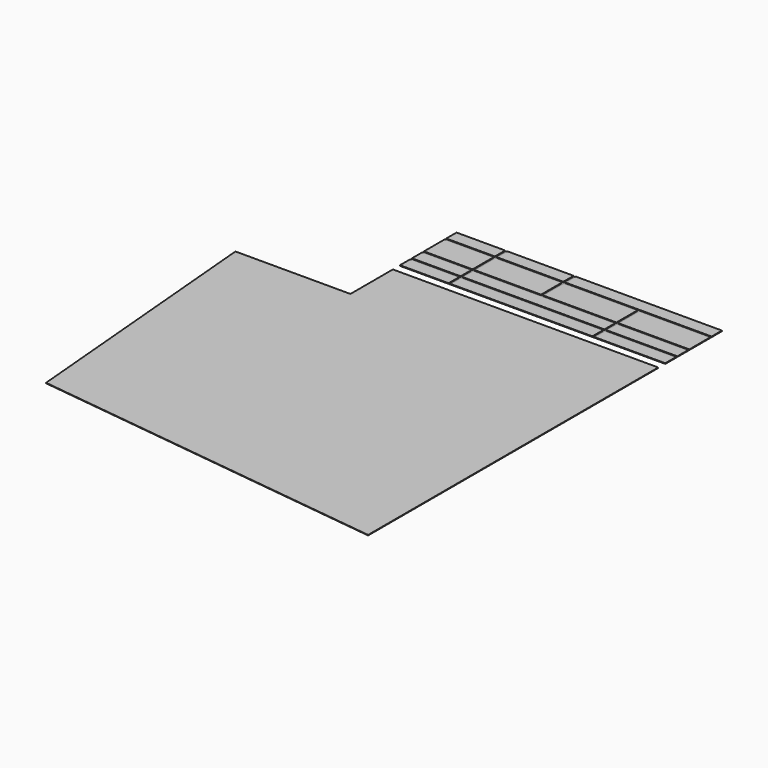
from build123d import *

# Parameters (mm, degrees)
F0_W     = 80100
F0_H     = 7280
F0_W_2   = 37500
F0_H_2   = 14560
F0_W_3   = 41400
F3_DEPTH = 25
F4_START = 280
F0_W_4   = 27500
F4_DEPTH = 70
F0_W_5   = 40000
F5_START = 280
F5_DEPTH = 70
F6_START = 280
F6_DEPTH = 70
F0_W_6   = 82600
F7_START = 280
F7_DEPTH = 70
F8_DEPTH = 280
F9_DEPTH = 280


# Not quite as in the source:
# - a feature names something its author has since deleted; it is built from what else it names


with BuildPart() as f3:
    # F0 (on Top) → F3 (new body)
    with BuildSketch(Plane.XY):
        Polygon((1151.0040283203, 20439.3217722573), (1151.0040283203, 27719.3217722572), (-48.9959716797, 27719.3217722572), (-48.9959716797, 20439.3217722573), (-37548.9959716797, 20439.3217722573), (-37548.9959716797, 27719.3217722572), (-38748.9959716797, 27719.3217722572), (-38748.9959716797, 20439.3217722573), (-66248.9959716797, 20439.3217722573), (-66248.9959716797, 19239.3217722572), (-38748.9959716797, 19239.3217722572), (-38748.9959716797, 4679.3217722572), (-66248.9959716797, 4679.3217722572), (-66248.9959716797, 3479.3217722572), (-38748.9959716797, 3479.3217722572), (-38748.9959716797, -3800.6782277428), (-66248.9959716797, -3800.6782277428), (-66248.9959716797, -5000.6782277428), (-38748.9959716797, -5000.6782277428), (-38748.9959716797, -12280.6782277428), (-37548.9959716797, -12280.6782277428), (-37548.9959716797, -5000.6782277428), (42551.0040283203, -5000.6782277428), (42551.0040283203, -12280.6782277428), (43751.0040283203, -12280.6782277428), (43751.0040283203, -5000.6782277428), (83751.0040283203, -5000.6782277428), (83751.0040283203, -3800.6782277427), (43751.0040283203, -3800.6782277427), (43751.0040283203, 3479.3217722572), (83751.0040283203, 3479.3217722572), (83751.0040283203, 4679.3217722573), (43751.0040283203, 4679.3217722573), (43751.0040283203, 19239.3217722572), (83751.0040283203, 19239.3217722573), (83751.0040283203, 20439.3217722573), align=None)
        with Locations((2501.0040283203, -160.6782277428)):
            Rectangle(F0_W, F0_H, mode=Mode.SUBTRACT)
        with Locations((-18798.9959716797, 11959.3217722572)):
            Rectangle(F0_W_2, F0_H_2, mode=Mode.SUBTRACT)
        with Locations((21851.0040283203, 11959.3217722572)):
            Rectangle(F0_W_3, F0_H_2, mode=Mode.SUBTRACT)
    extrude(amount=F3_DEPTH)


with BuildPart() as f4:
    # F0 (on Top) → F4 (new body)
    with BuildSketch(Plane.XY.offset(F4_START)):
        with Locations((-52498.9959716797, -8640.6782277428)):
            Rectangle(F0_W_4, F0_H)
    extrude(amount=F4_DEPTH)


with BuildPart() as f4b:
    # F0 (on Top) → F4, piece 2 (new body)
    with BuildSketch(Plane.XY.offset(F4_START)):
        with Locations((-18798.9959716797, 24079.3217722572)):
            Rectangle(F0_W_2, F0_H)
    extrude(amount=F4_DEPTH)


with BuildPart() as f4c:
    # F0 (on Top) → F4, piece 3 (new body)
    with BuildSketch(Plane.XY.offset(F4_START)):
        with Locations((63751.0040283203, 11959.3217722573)):
            Rectangle(F0_W_5, F0_H_2)
    extrude(amount=F4_DEPTH)


with BuildPart() as f5:
    # F0 (on Top) → F5 (new body)
    with BuildSketch(Plane.XY.offset(F5_START)):
        with Locations((2501.0040283203, -8640.6782277428)):
            Rectangle(F0_W, F0_H)
    extrude(amount=F5_DEPTH)


with BuildPart() as f5b:
    # F0 (on Top) → F5, piece 2 (new body)
    with BuildSketch(Plane.XY.offset(F5_START)):
        with Locations((-52498.9959716797, 24079.3217722572)):
            Rectangle(F0_W_4, F0_H)
    extrude(amount=F5_DEPTH)


with BuildPart() as f6:
    # F0 (on Top) → F6 (new body)
    with BuildSketch(Plane.XY.offset(F6_START)):
        with Locations((2501.0040283203, -160.6782277428)):
            Rectangle(F0_W, F0_H)
    extrude(amount=F6_DEPTH)


with BuildPart() as f6b:
    # F0 (on Top) → F6, piece 2 (new body)
    with BuildSketch(Plane.XY.offset(F6_START)):
        with Locations((42451.0040283203, 24079.3217722573)):
            Rectangle(F0_W_6, F0_H)
    extrude(amount=F6_DEPTH)


with BuildPart() as f7:
    # F0 (on Top) → F7 (new body)
    with BuildSketch(Plane.XY.offset(F7_START)):
        with Locations((63751.0040283203, -8640.6782277428)):
            Rectangle(F0_W_5, F0_H)
    extrude(amount=F7_DEPTH)


with BuildPart() as f7b:
    # F0 (on Top) → F7, piece 2 (new body)
    with BuildSketch(Plane.XY.offset(F7_START)):
        with Locations((63751.0040283203, -160.6782277427)):
            Rectangle(F0_W_5, F0_H)
    extrude(amount=F7_DEPTH)


with BuildPart() as f7c:
    # F0 (on Top) → F7, piece 3 (new body)
    with BuildSketch(Plane.XY.offset(F7_START)):
        with Locations((21851.0040283203, 11959.3217722573)):
            Rectangle(F0_W_3, F0_H_2)
    extrude(amount=F7_DEPTH)


with BuildPart() as f7d:
    # F0 (on Top) → F7, piece 4 (new body)
    with BuildSketch(Plane.XY.offset(F7_START)):
        with Locations((-18798.9959716797, 11959.3217722572)):
            Rectangle(F0_W_2, F0_H_2)
    extrude(amount=F7_DEPTH)


with BuildPart() as f7e:
    # F0 (on Top) → F7, piece 5 (new body)
    with BuildSketch(Plane.XY.offset(F7_START)):
        with Locations((-52498.9959716797, 11959.3217722572)):
            Rectangle(F0_W_4, F0_H_2)
    extrude(amount=F7_DEPTH)


with BuildPart() as f7f:
    # F0 (on Top) → F7, piece 6 (new body)
    with BuildSketch(Plane.XY.offset(F7_START)):
        with Locations((-52498.9959716797, -160.6782277428)):
            Rectangle(F0_W_4, F0_H)
    extrude(amount=F7_DEPTH)


with BuildPart() as f8:
    # F0 (on Top) → F8 (new body)
    with BuildSketch(Plane.XY):
        with Locations((42451.0040283203, 24079.3217722573)):
            Rectangle(F0_W_6, F0_H)
    extrude(amount=F8_DEPTH)


with BuildPart() as f8b:
    # F0 (on Top) → F8, piece 2 (new body)
    with BuildSketch(Plane.XY):
        with Locations((63751.0040283203, 11959.3217722573)):
            Rectangle(F0_W_5, F0_H_2)
    extrude(amount=F8_DEPTH)


with BuildPart() as f8c:
    # F0 (on Top) → F8, piece 3 (new body)
    with BuildSketch(Plane.XY):
        with Locations((21851.0040283203, 11959.3217722573)):
            Rectangle(F0_W_3, F0_H_2)
    extrude(amount=F8_DEPTH)


with BuildPart() as f8d:
    # F0 (on Top) → F8, piece 4 (new body)
    with BuildSketch(Plane.XY):
        with Locations((-18798.9959716797, 24079.3217722572)):
            Rectangle(F0_W_2, F0_H)
    extrude(amount=F8_DEPTH)


with BuildPart() as f8e:
    # F0 (on Top) → F8, piece 5 (new body)
    with BuildSketch(Plane.XY):
        with Locations((-52498.9959716797, 24079.3217722572)):
            Rectangle(F0_W_4, F0_H)
    extrude(amount=F8_DEPTH)


with BuildPart() as f8f:
    # F0 (on Top) → F8, piece 6 (new body)
    with BuildSketch(Plane.XY):
        with Locations((-52498.9959716797, 11959.3217722572)):
            Rectangle(F0_W_4, F0_H_2)
    extrude(amount=F8_DEPTH)


with BuildPart() as f8g:
    # F0 (on Top) → F8, piece 7 (new body)
    with BuildSketch(Plane.XY):
        with Locations((-52498.9959716797, -160.6782277428)):
            Rectangle(F0_W_4, F0_H)
    extrude(amount=F8_DEPTH)


with BuildPart() as f8h:
    # F0 (on Top) → F8, piece 8 (new body)
    with BuildSketch(Plane.XY):
        with Locations((-52498.9959716797, -8640.6782277428)):
            Rectangle(F0_W_4, F0_H)
    extrude(amount=F8_DEPTH)


with BuildPart() as f8i:
    # F0 (on Top) → F8, piece 9 (new body)
    with BuildSketch(Plane.XY):
        with Locations((2501.0040283203, -8640.6782277428)):
            Rectangle(F0_W, F0_H)
    extrude(amount=F8_DEPTH)


with BuildPart() as f8j:
    # F0 (on Top) → F8, piece 10 (new body)
    with BuildSketch(Plane.XY):
        with Locations((2501.0040283203, -160.6782277428)):
            Rectangle(F0_W, F0_H)
    extrude(amount=F8_DEPTH)


with BuildPart() as f8k:
    # F0 (on Top) → F8, piece 11 (new body)
    with BuildSketch(Plane.XY):
        with Locations((63751.0040283203, -160.6782277427)):
            Rectangle(F0_W_5, F0_H)
    extrude(amount=F8_DEPTH)


with BuildPart() as f8l:
    # F0 (on Top) → F8, piece 12 (new body)
    with BuildSketch(Plane.XY):
        with Locations((63751.0040283203, -8640.6782277428)):
            Rectangle(F0_W_5, F0_H)
    extrude(amount=F8_DEPTH)


with BuildPart() as f8m:
    # F0 (on Top) → F8, piece 13 (new body)
    with BuildSketch(Plane.XY):
        with Locations((-18798.9959716797, 11959.3217722572)):
            Rectangle(F0_W_2, F0_H_2)
    extrude(amount=F8_DEPTH)


with BuildPart() as f9:
    # F2 (on Top) → F9 (new body)
    with BuildSketch(Plane.XY):
        Polygon((83751.0040283203, -17280.6782277427), (-66248.9959716797, -17280.6782277428), (-66248.9959716797, -47280.6782277428), (-131248.9959716797, -47280.6782277428), (-118106.8892489593, -197495.6454369067), (83751.0040283203, -222280.6782277427), align=None)
    extrude(amount=F9_DEPTH)


solid = Compound([f3.part, f4.part, f4b.part, f4c.part, f5.part, f5b.part, f6.part, f6b.part, f7.part, f7b.part, f7c.part, f7d.part, f7e.part, f7f.part, f8.part, f8b.part, f8c.part, f8d.part, f8e.part, f8f.part, f8g.part, f8h.part, f8i.part, f8j.part, f8k.part, f8l.part, f8m.part, f9.part])
